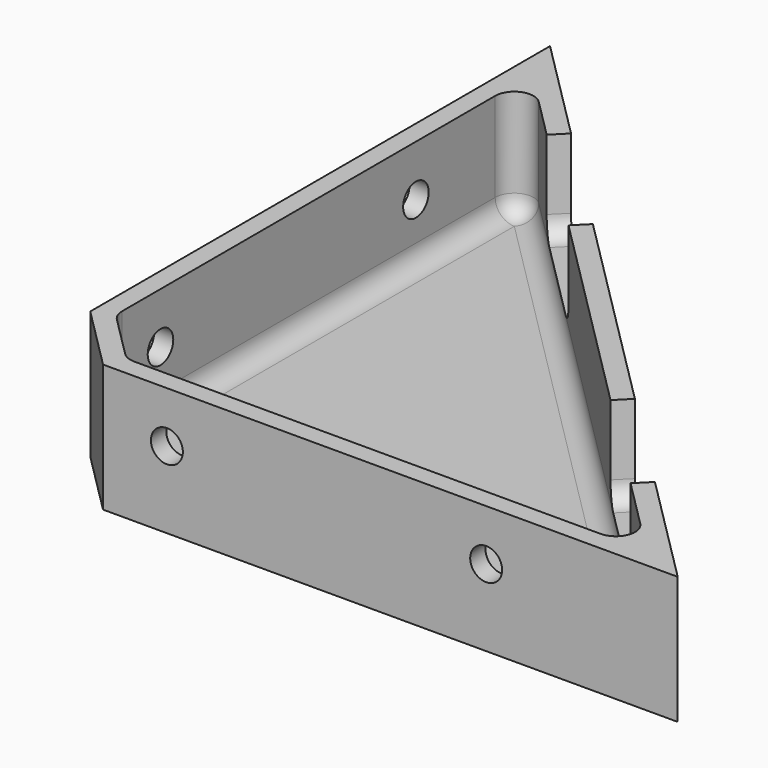
from build123d import *

# Parameters (mm, degrees)
F1_DEPTH  = 20
F2_SIZE   = 10
F3_T      = -3
F5_R      = 2.5
F6_DEPTH  = 3
F4_R      = 2.5
F7_DEPTH  = 3
F9_R      = 3
F10_DEPTH = 3


with BuildPart() as f1:
    # F0 (on Top) → F1 (new body)
    with BuildSketch(Plane.XY):
        Polygon((0, 100), (0, 0), (100, 0), align=None)
    extrude(amount=F1_DEPTH)

    # F2
    f2_edges = [f1.edges().sort_by_distance(p)[0] for p in [
        (0, 0, 10),
    ]]
    chamfer(f2_edges, length=F2_SIZE)

    # F3
    f3_openings = [f1.faces().sort_by_distance(p)[0] for p in [
        (33.636364, 33.636364, 20),
    ]]
    offset(amount=F3_T, openings=f3_openings)

    # F5 (on Front) → F6 (cut, through all)
    with BuildSketch(Plane.XZ):
        with Locations((20, 12)):
            Circle(F5_R)
        with Locations((70, 12)):
            Circle(F5_R)
    extrude(amount=-F6_DEPTH, mode=Mode.SUBTRACT)

    # F4 (on Right) → F7 (cut, through all)
    with BuildSketch(Plane.YZ):
        with Locations((20, 12)):
            Circle(F4_R)
        with Locations((70, 12)):
            Circle(F4_R)
    extrude(amount=F7_DEPTH, mode=Mode.SUBTRACT)

    # F9
    f9_edges = [f1.edges().sort_by_distance(p)[0] for p in [
        (3, 52, 3),
        (52, 3, 3),
        (92.757359, 3, 11.5),
        (3, 92.757359, 11.5),
        (47.87868, 47.87868, 3),
        (3, 11.242641, 11.5),
        (11.242641, 3, 11.5),
    ]]
    fillet(f9_edges, radius=F9_R)

    # F8 (on face) → F10 (cut, through all)
    with BuildSketch(Plane(origin=(50, 50, 0), x_dir=(-0.7071067812, 0.7071067812, 0), z_dir=(0.7071067812, 0.7071067812, 0))):
        with BuildLine():
            Line((-23.2842712475, 20), (-45.4264068712, 20))
            Line((-45.4264068712, 20), (-45.4264068712, 9))
            ThreePointArc((-45.4264068712, 9), (-44.5477272148, 6.8786796564), (-42.4264068712, 6))
            Line((-42.4264068712, 6), (-26.2842712475, 6))
            ThreePointArc((-26.2842712475, 6), (-24.1629509039, 6.8786796564), (-23.2842712475, 9))
            Line((-23.2842712475, 9), (-23.2842712475, 20))
        make_face()
        with BuildLine():
            Line((47.4264068712, 20), (23.2842712475, 20))
            Line((23.2842712475, 20), (23.2842712475, 9))
            ThreePointArc((23.2842712475, 9), (24.1629509039, 6.8786796564), (26.2842712475, 6))
            Line((26.2842712475, 6), (44.4264068712, 6))
            ThreePointArc((44.4264068712, 6), (46.5477272148, 6.8786796564), (47.4264068712, 9))
            Line((47.4264068712, 9), (47.4264068712, 20))
        make_face()
    extrude(amount=-F10_DEPTH, mode=Mode.SUBTRACT)


solid = f1.part
